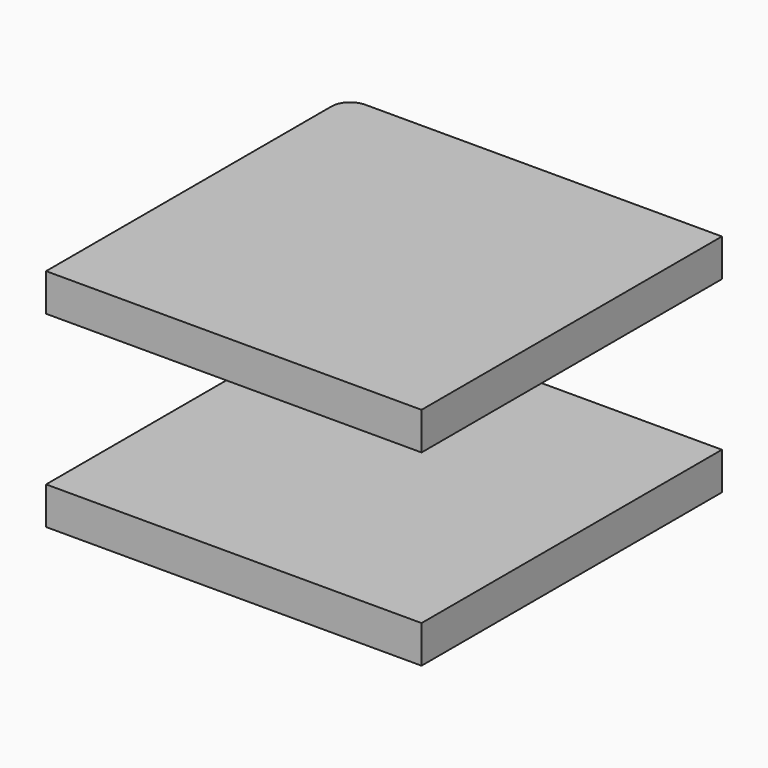
from build123d import *

# Parameters (mm, degrees)
F0_W      = 100
F0_H      = 100
F1_DEPTH  = 60
F3_START  = -10
F1_FACE_W = 100
F1_FACE_H = 100
F3_DEPTH  = 40
F4_R      = 5


with BuildPart() as f1:
    # F0 (on Top) → F1 (new body)
    with BuildSketch(Plane.XY):
        Rectangle(F0_W, F0_H)
    extrude(amount=F1_DEPTH)

    # F1_face (on face) → F3 (cut)
    with BuildSketch(Plane.XY.offset(60).offset(F3_START)):
        Rectangle(F1_FACE_W, F1_FACE_H)
    extrude(amount=-F3_DEPTH, mode=Mode.SUBTRACT)

    # F4
    f4_edges = [f1.edges().sort_by_distance(p)[0] for p in [
        (-50, 50, 5),
        (-50, 50, 55),
    ]]
    fillet(f4_edges, radius=F4_R)


solid = f1.part
